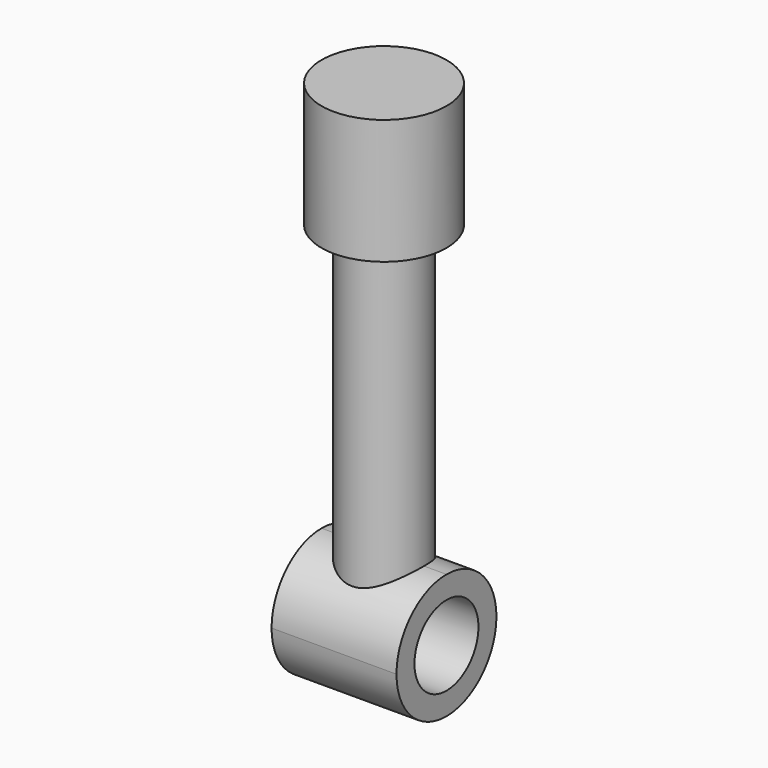
from build123d import *

# Parameters (mm, degrees)
F0_R         = 2.54
F1_DEPTH     = 18.25625
F2_W         = 7.9375
F2_H         = 7.9375
F3_DEPTH     = 7.9375
F4_R         = 3.96875
F5_DEPTH     = 7.9375
F6_T1_DEPTH  = 27.78125
F6_T6_DEPTH  = 27.78125
F6_S7_R      = 2.54
F6_T8_DEPTH  = 16
F6_T12_DEPTH = 27.78125
F6_S13_R     = 2.54
F6_T14_DEPTH = 16
F7_R         = 2.54
F8_DEPTH     = 7.9375


# Not quite as in the source:
# - a fillet or chamfer that OpenCascade refuses, or shapes differently, is made with other operations: its cross-section is extruded or revolved along the edge and cut away or added


with BuildPart() as f1:
    # F0 (on Top) → F1 (new body)
    with BuildSketch(Plane.XY):
        Circle(F0_R)
    extrude(amount=F1_DEPTH)

    # F2 (on face) → F3 (join)
    with BuildSketch(Plane(origin=(0, 0, 0), x_dir=(1, 0, 0), z_dir=(0, 0, -1))):
        Rectangle(F2_W, F2_H)
    extrude(amount=F3_DEPTH)

    # F4 (on face) → F5 (join)
    with BuildSketch(Plane.XY.offset(18.25625)):
        Circle(F4_R)
    extrude(amount=F5_DEPTH)

    # F6: fillet of radius 3.96875 on 4 edges, made by hand

    # F6_s2 → F6_t1 (cut)
    with BuildSketch(Plane.YZ.offset(-13.890625)):
        with BuildLine():
            ThreePointArc((3.96875, -3.96875), (2.8063300378, -6.7750800378), (0, -7.9375))
            Line((0, -7.9375), (3.96875, -7.9375))
            Line((3.96875, -7.9375), (3.96875, -3.96875))
        make_face()
        with BuildLine():
            ThreePointArc((-3.96875, -3.96875), (-2.8063300378, -6.7750800378), (0, -7.9375))
            Line((0, -7.9375), (-3.96875, -7.9375))
            Line((-3.96875, -7.9375), (-3.96875, -3.96875))
        make_face()
    extrude(amount=F6_T1_DEPTH, mode=Mode.SUBTRACT)


with BuildPart() as f6_tool4:
    # F6_s5 → F6_t6 (new body)
    with BuildSketch(Plane.YZ.offset(13.890625)):
        with BuildLine():
            ThreePointArc((0, 0), (-2.8063300378, -1.1624199622), (-3.96875, -3.96875))
            Line((-3.96875, -3.96875), (-3.96875, 0))
            Line((-3.96875, 0), (0, 0))
        make_face()
    extrude(amount=-F6_T6_DEPTH)

    # F6_s7 → F6_t8 (cut, symmetric)
    with BuildSketch(Plane.XY.offset(-2)):
        Circle(F6_S7_R)
    extrude(amount=F6_T8_DEPTH, both=True, mode=Mode.SUBTRACT)


with BuildPart() as f1_1:
    add(f1.part)

    # F6_t3: cut F6_tool4
    add(f6_tool4.part, mode=Mode.SUBTRACT)


with BuildPart() as f6_tool10:
    # F6_s11 → F6_t12 (new body)
    with BuildSketch(Plane.YZ.offset(-13.890625)):
        with BuildLine():
            ThreePointArc((0, 0), (2.8063300378, -1.1624199622), (3.96875, -3.96875))
            Line((3.96875, -3.96875), (3.96875, 0))
            Line((3.96875, 0), (0, 0))
        make_face()
    extrude(amount=F6_T12_DEPTH)

    # F6_s13 → F6_t14 (cut, symmetric)
    with BuildSketch(Plane.XY.offset(-2)):
        Circle(F6_S13_R)
    extrude(amount=F6_T14_DEPTH, both=True, mode=Mode.SUBTRACT)


with BuildPart() as f1_2:
    add(f1_1.part)

    # F6_t9: cut F6_tool10
    add(f6_tool10.part, mode=Mode.SUBTRACT)

    # F7 (on face) → F8 (cut, through all)
    with BuildSketch(Plane(origin=(-3.96875, 0, 0), x_dir=(0, -1, 0), z_dir=(-1, 0, 0))):
        with Locations((0, -3.96875)):
            Circle(F7_R)
    extrude(amount=-F8_DEPTH, mode=Mode.SUBTRACT)


solid = f1_2.part
